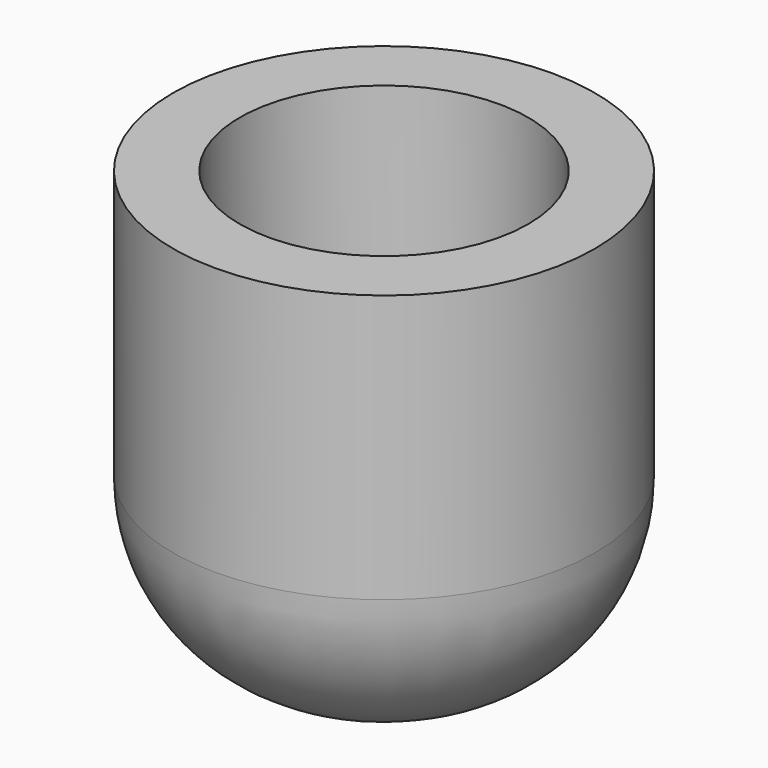
from build123d import *

# Parameters (mm, degrees)
F0_R     = 6.5
F0_R_2   = 2.5
F1_DEPTH = 3
F0_R_3   = 9.5
F2_DEPTH = 20


# Not quite as in the source:
# - a fillet or chamfer that OpenCascade refuses, or shapes differently, is made with other operations: its cross-section is extruded or revolved along the edge and cut away or added


with BuildPart() as f1:
    # F0 (on Top) → F1 (new body)
    with BuildSketch(Plane.XY):
        Circle(F0_R)
        Circle(F0_R_2, mode=Mode.SUBTRACT)
    extrude(amount=F1_DEPTH)

    # F0 (on Top) → F2 (join)
    with BuildSketch(Plane.XY):
        Circle(F0_R_3)
        Circle(F0_R, mode=Mode.SUBTRACT)
    extrude(amount=F2_DEPTH)

    # F3: fillet of radius 8 on 1 edges, made by hand

    # F3_s1 → F3_t2 (revolve, cut)
    with BuildSketch(Plane.XZ):
        with BuildLine():
            ThreePointArc((2.5, 0), (7.5, 2.6457513111), (9.5, 7.9372539332))
            Line((9.5, 7.9372539332), (9.5, 0))
            Line((9.5, 0), (2.5, 0))
        make_face()
    revolve(axis=Axis((0, 0, 0), (0, 0, 1)), mode=Mode.SUBTRACT)

    # F4 (on Right) → F5 (revolve)
    with BuildSketch(Plane.YZ):
        Polygon((7.5, 13), (2, 3), (7.5, 3), align=None)
    revolve(axis=Axis((0, 0, 1.5), (0, 0, 1)))


solid = f1.part
